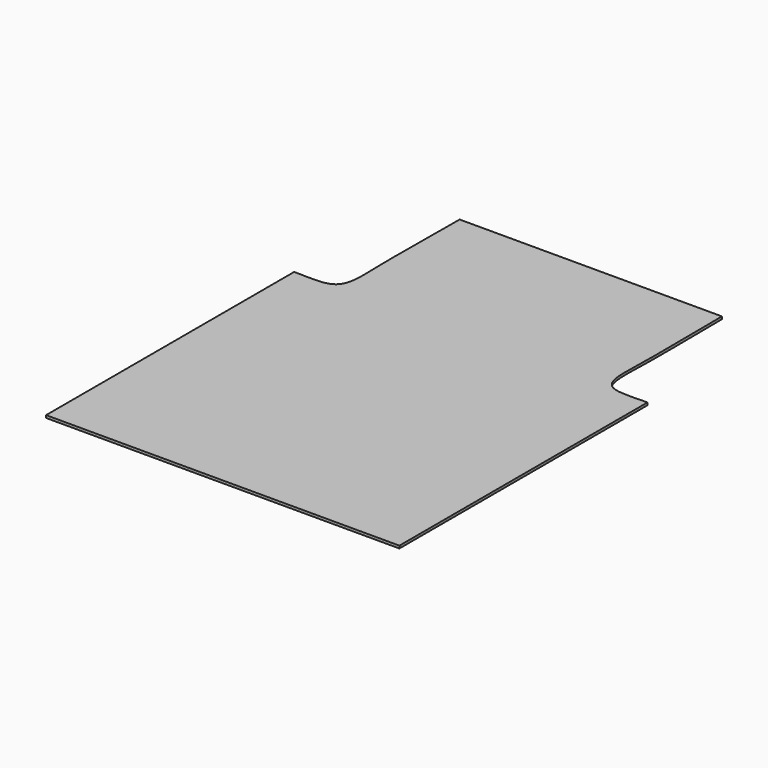
from build123d import *

# Parameters (mm, degrees)
F0_W     = 697.0556974411
F0_H     = 1815.3920248151
F1_DEPTH = 10
F3_DEPTH = 660


with BuildPart() as f1:
    # F0 (on Top) → F1 (new body)
    with BuildSketch(Plane.XY):
        with Locations((348.5278487206, 992.8541146219)):
            Rectangle(F0_W, F0_H)
    extrude(amount=-F1_DEPTH)

    # F2 (on face) → F3 (cut)
    with BuildSketch(Plane.XY):
        with BuildLine():
            add(Edge.make_bspline(
                [(518.803774091, 2038.8926588478), (514.4141140373, 1900.5501270294), (527.0135085035, 1534.9048792953), (504.258722184, 1284.8443561216), (652.2567457375, 1310.686684836), (731.5574045275, 1309.2447331839)],
                knots=[0, 0, 0, 0, 0.4528842523, 0.7287221415, 1, 1, 1, 1], degree=3))
            Line((731.5574045275, 1309.2447331839), (731.5574045275, 2029.0073490817))
            Line((731.5574045275, 2029.0073490817), (518.803774091, 2038.8926588478))
        make_face()
    extrude(amount=-F3_DEPTH, mode=Mode.SUBTRACT)

    # F4: F1 across plane


with BuildPart() as f1_1:
    add(f1.part)
    add(f1.part.mirror(Plane.YZ))


solid = f1_1.part
